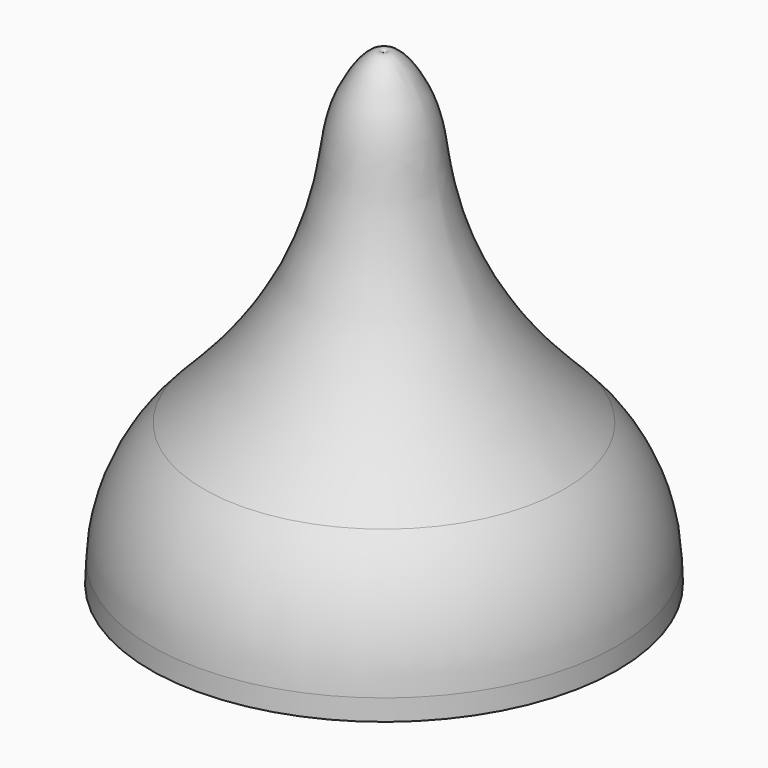
from build123d import *


with BuildPart() as f1:
    # F0 (on Front) → F1 (revolve)
    with BuildSketch(Plane.XZ):
        with BuildLine():
            add(Edge.make_bspline(
                [(19.6185046924, 15.4489545738), (18.0615910097, 17.0393280025), (9.8841190577, 25.6741635963), (5.2688794872, 38.1624367236), (5.3021085915, 46.3445011141), (0.9578001157, 51.9446241181), (0, 50.8)],
                knots=[0.6543608934, 0.6543608934, 0.6543608934, 0.6543608934, 0.6874668641, 0.8325923374, 0.9268519331, 1, 1, 1, 1], degree=3))
            Line((0, 50.8), (0, 41.2659347057))
            Line((0, 41.2659347057), (2.8961050237, 32.7684234659))
            add(Edge.make_bspline(
                [(2.8961050237, 32.7684234659), (3.0541790872, 32.3306892834), (3.2067470899, 31.88093585), (3.3519621793, 31.4308851957)],
                knots=[0.1125349186, 0.1125349186, 0.1125349186, 0.1125349186, 0.1322894717, 0.1322894717, 0.1322894717, 0.1322894717], degree=3))
            add(Edge.make_bspline(
                [(3.3519621793, 31.4308851957), (4.8894737939, 26.6658286799), (6.2695761916, 17.3810267229), (14.6603033782, 4.5264494367), (13.3471656591, 3.0574093107)],
                knots=[0.1322894717, 0.1322894717, 0.1322894717, 0.1322894717, 0.3414471766, 0.5370072443, 0.5370072443, 0.5370072443, 0.5370072443], degree=3))
            add(Edge.make_bspline(
                [(13.3471656591, 3.0574093107), (12.9263416093, 2.5866228836), (11.9542577346, 2.602882575), (10.7055676901, 3.0574093107)],
                knots=[0.5370072443, 0.5370072443, 0.5370072443, 0.5370072443, 0.5996787969, 0.5996787969, 0.5996787969, 0.5996787969], degree=3))
            Line((10.7055676901, 3.0574093107), (2.7245637711, 3.0574093107))
            add(Edge.make_bspline(
                [(2.7245637711, 3.0574093107), (2.6912612106, 1.2251085712), (2.3423176425, 0.9234684917), (2.7529783998, 0.0706794419), (2.7902495499, 0)],
                knots=[0.2225094867, 0.2225094867, 0.2225094867, 0.2225094867, 0.2763140985, 0.2809425098, 0.2809425098, 0.2809425098, 0.2809425098], degree=3))
            Line((2.7902495499, 0), (25.4, 0))
            Line((25.4, 0), (25.3112478254, 2.2472257004))
            ThreePointArc((25.3112478254, 2.2472257004), (23.6921242971, 9.3772941458), (19.6185046924, 15.4489545738))
        make_face()
        with BuildLine():
            add(Edge.make_bspline(
                [(2.8961050237, 32.7684234659), (3.0541790872, 32.3306892834), (3.2067470899, 31.88093585), (3.3519621793, 31.4308851957)],
                knots=[0.1125349186, 0.1125349186, 0.1125349186, 0.1125349186, 0.1322894717, 0.1322894717, 0.1322894717, 0.1322894717], degree=3))
            Line((2.8961050237, 32.7684234659), (3.3519621793, 31.4308851957))
        make_face()
        with BuildLine():
            Line((0, 0), (2.7902495499, 0))
            add(Edge.make_bspline(
                [(2.7245637711, 3.0574093107), (2.6912612106, 1.2251085712), (2.3423176425, 0.9234684917), (2.7529783998, 0.0706794419), (2.7902495499, 0)],
                knots=[0.2225094867, 0.2225094867, 0.2225094867, 0.2225094867, 0.2763140985, 0.2809425098, 0.2809425098, 0.2809425098, 0.2809425098], degree=3))
            Line((2.7245637711, 3.0574093107), (0, 3.0574093107))
            Line((0, 3.0574093107), (0, 0))
        make_face()
        with BuildLine():
            Line((13.3471656591, 3.0574093107), (10.7055676901, 3.0574093107))
            add(Edge.make_bspline(
                [(13.3471656591, 3.0574093107), (12.9263416093, 2.5866228836), (11.9542577346, 2.602882575), (10.7055676901, 3.0574093107)],
                knots=[0.5370072443, 0.5370072443, 0.5370072443, 0.5370072443, 0.5996787969, 0.5996787969, 0.5996787969, 0.5996787969], degree=3))
        make_face()
    revolve(axis=Axis((0, 0, 1.5287046554), (0, 0, -1)))


solid = f1.part
